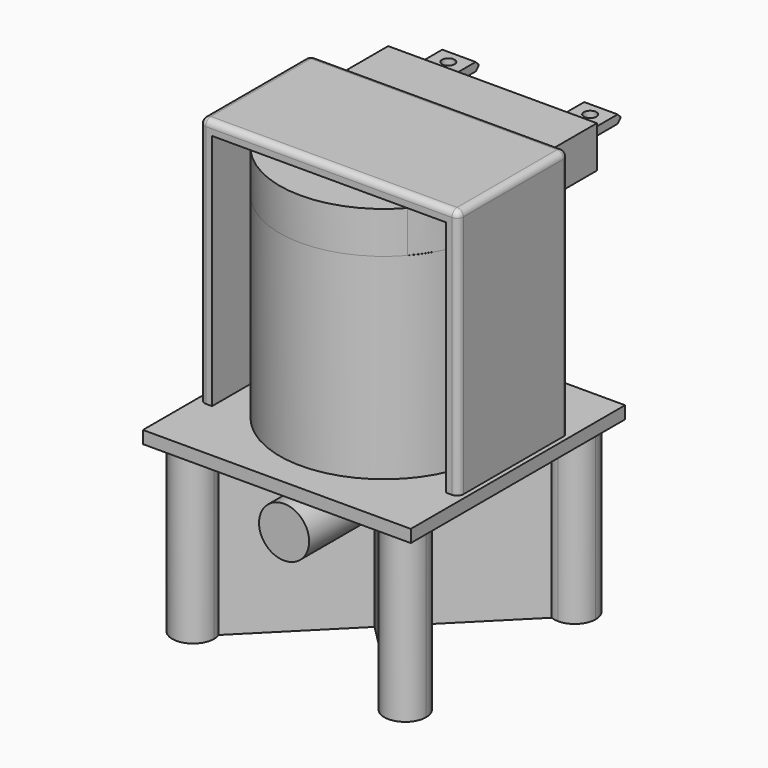
from build123d import *

# Parameters (mm, degrees)
F0_W      = 31
F0_H      = 16.5
F1_DEPTH  = 30
F2_W      = 28
F2_H      = 28.5
F3_DEPTH  = 16.5
F4_R      = 0.762
F5_W      = 28
F5_H      = 24.4999924
F6_DEPTH  = 5
F7_R      = 12.4999974
F8_DEPTH  = 23.5
F10_DEPTH = 5
F11_W     = 2
F11_H     = 0.5
F12_DEPTH = 6
F13_R     = 0.75
F14_DEPTH = 1
F15_SIZE  = 0.4
F16_SIZE  = 0.4
F18_DEPTH = 5
F19_W     = 32.0802
F19_H     = 32.0802
F20_DEPTH = 1.5
F22_DEPTH = 20
F26_DEPTH = 20
F27_R     = 3
F28_DEPTH = 31


# Not quite as in the source:
# - a feature of the source that left no trace in its solid (it failed there, or was rolled back) is left out


with BuildPart() as f1:
    # F0 (on Top) → F1 (new body)
    with BuildSketch(Plane.XY):
        Rectangle(F0_W, F0_H)
    extrude(amount=F1_DEPTH)

    # F2 (on face) → F3 (cut, through all)
    with BuildSketch(Plane.XZ.offset(8.25)):
        with Locations((0, 14.25)):
            Rectangle(F2_W, F2_H)
    extrude(amount=-F3_DEPTH, mode=Mode.SUBTRACT)

    # F4
    f4_edges = [f1.edges().sort_by_distance(p)[0] for p in [
        (15.5, 8.25, 15),
        (0, 8.25, 30),
        (-15.5, 8.25, 15),
        (15.5, 0, 30),
        (15.5, -8.25, 15),
        (0, -8.25, 30),
        (-15.5, 0, 30),
        (-15.5, -8.25, 15),
    ]]
    fillet(f4_edges, radius=F4_R)

    # F5 (on face) → F6 (join)
    with BuildSketch(Plane(origin=(0, 0, 28.5), x_dir=(1, 0, 0), z_dir=(0, 0, -1))):
        with Locations((0, -3.9999962)):
            Rectangle(F5_W, F5_H)
    extrude(amount=F6_DEPTH)

    # F7 (on face) → F8 (join)
    with BuildSketch(Plane(origin=(0, 0, 23.5), x_dir=(1, 0, 0), z_dir=(0, 0, -1))):
        Circle(F7_R)
    extrude(amount=F8_DEPTH)

    # F9 (on face) → F10 (cut)
    with BuildSketch(Plane(origin=(0, 0, 23.5), x_dir=(1, 0, 0), z_dir=(0, 0, -1))):
        with BuildLine():
            add(Edge.make_bspline(
                [(9.3908165247, 8.25), (9.9761542333, 7.5152910471), (11.2114839399, 5.7745359804), (12.1932801678, 3.3671524419), (12.4792695901, 0.7813469518), (12.4999974, 0)],
                knots=[0, 0, 0, 0, 0.3330931337, 0.6537874323, 1, 1, 1, 1], degree=3))
            Line((12.4999974, 0), (12.4999974, -16.2499924))
            Line((12.4999974, -16.2499924), (14, -16.2499924))
            Line((14, -16.2499924), (14, 8.25))
            Line((14, 8.25), (9.3908165247, 8.25))
        make_face()
        with BuildLine():
            add(Edge.make_bspline(
                [(-9.3908165247, 8.25), (-9.8951466827, 7.6039833324), (-10.9690015511, 6.2442324236), (-12.2412171784, 3.3192353758), (-12.4077121811, 1.117573176), (-12.4999974, 0)],
                knots=[0, 0, 0, 0, 0.3063307587, 0.6473537439, 1, 1, 1, 1], degree=3))
            Line((-9.3908165247, 8.25), (-14, 8.25))
            Line((-14, 8.25), (-14, -16.2499924))
            Line((-14, -16.2499924), (-12.4999974, -16.2499924))
            Line((-12.4999974, -16.2499924), (-12.4999974, 0))
        make_face()
    extrude(amount=-F10_DEPTH, mode=Mode.SUBTRACT)

    # F11 (on face) → F12 (join)
    with BuildSketch(Plane(origin=(0, 16.2499924, 0), x_dir=(-1, 0, 0), z_dir=(0, 1, 0))):
        with Locations((-7.4999974, 25.75)):
            Rectangle(F11_W, F11_H)
        with Locations((-7.4999974, 26.25)):
            Rectangle(F11_W, F11_H)
        with Locations((9.4999974, 25.75)):
            Rectangle(F11_W, F11_H)
        with Locations((7.4999974, 25.75)):
            Rectangle(F11_W, F11_H)
        with Locations((9.4999974, 26.25)):
            Rectangle(F11_W, F11_H)
        with Locations((7.4999974, 26.25)):
            Rectangle(F11_W, F11_H)
        with Locations((-9.4999974, 25.75)):
            Rectangle(F11_W, F11_H)
        with Locations((-9.4999974, 26.25)):
            Rectangle(F11_W, F11_H)
    extrude(amount=F12_DEPTH)

    # F13 (on face) → F14 (cut, through all)
    with BuildSketch(Plane.XY.offset(26.5)):
        with Locations((8.4999974, 20.2499924)):
            Circle(F13_R)
        with Locations((-8.4999974, 20.2499924)):
            Circle(F13_R)
    extrude(amount=-F14_DEPTH, mode=Mode.SUBTRACT)

    # F15
    f15_edges = [f1.edges().sort_by_distance(p)[0] for p in [
        (8.499997, 22.249992, 26.5),
        (-8.499997, 22.249992, 26.5),
    ]]
    chamfer(f15_edges, length=F15_SIZE)

    # F16
    f16_edges = [f1.edges().sort_by_distance(p)[0] for p in [
        (8.499997, 22.249992, 25.5),
        (-8.499997, 22.249992, 25.5),
    ]]
    chamfer(f16_edges, length=F16_SIZE)

    # F17 (on face) → F18 (join)
    with BuildSketch(Plane.XY.offset(23.5)):
        with BuildLine():
            Line((9.3908165247, -8.25), (-9.3908165247, -8.25))
            ThreePointArc((-9.3908165247, -8.25), (0, -12.4999974), (9.3908165247, -8.25))
        make_face()
    extrude(amount=F18_DEPTH)

    # F19 (on face) → F20 (join)
    with BuildSketch(Plane(origin=(0, 0, 0), x_dir=(1, 0, 0), z_dir=(0, 0, -1))):
        Rectangle(F19_W, F19_H)
    extrude(amount=F20_DEPTH)

    # F21 (on face) → F22 (join)
    with BuildSketch(Plane(origin=(0, 0, -1.5), x_dir=(1, 0, 0), z_dir=(0, 0, -1))):
        with BuildLine():
            ThreePointArc((-10.2, -12.7), (-10.932233047, -10.932233047), (-12.7, -10.2))
            ThreePointArc((-12.7, -10.2), (-14.467766953, -14.467766953), (-10.2, -12.7))
        make_face()
        with BuildLine():
            ThreePointArc((-12.7, 10.2), (-10.932233047, 10.932233047), (-10.2, 12.7))
            ThreePointArc((-10.2, 12.7), (-14.467766953, 14.467766953), (-12.7, 10.2))
        make_face()
        with BuildLine():
            ThreePointArc((12.7, 10.2), (14.467766953, 10.932233047), (15.2, 12.7))
            ThreePointArc((15.2, 12.7), (12.7, 15.2), (10.2, 12.7))
            ThreePointArc((10.2, 12.7), (10.932233047, 10.932233047), (12.7, 10.2))
        make_face()
        with BuildLine():
            ThreePointArc((15.2, -12.7), (14.467766953, -10.932233047), (12.7, -10.2))
            ThreePointArc((12.7, -10.2), (10.932233047, -10.932233047), (10.2, -12.7))
            ThreePointArc((10.2, -12.7), (12.7, -15.2), (15.2, -12.7))
        make_face()
    extrude(amount=F22_DEPTH)


with BuildPart() as f26:
    # F25 (on face) → F26 (new body)
    with BuildSketch(Plane(origin=(0, 0, -21.5), x_dir=(1, 0, 0), z_dir=(0, 0, -1))):
        with BuildLine():
            ThreePointArc((-11.7690392124, -10.379803454), (-10.9186518108, -10.945919435), (-10.3657199255, -11.8049376927))
            Line((-10.3657199255, -11.8049376927), (-3.5923e-06, -1.4158147652))
            Line((-3.5923e-06, -1.4158147652), (1.4126173591, -4.0058e-06))
            Line((1.4126173591, -4.0058e-06), (11.7690392124, 10.379803454))
            ThreePointArc((11.7690392124, 10.379803454), (10.9186518108, 10.945919435), (10.3657199255, 11.8049376927))
            Line((10.3657199255, 11.8049376927), (0, 1.4158111649))
            Line((0, 1.4158111649), (-1.4126177626, 3.6014e-06))
            Line((-1.4126177626, 3.6014e-06), (-11.7690392124, -10.379803454))
        make_face()
        with BuildLine():
            Line((1.4126173591, -4.0058e-06), (-3.5923e-06, -1.4158147652))
            Line((-3.5923e-06, -1.4158147652), (10.3664711716, -11.8029809328))
            ThreePointArc((10.3664711716, -11.8029809328), (10.9201168847, -10.9444328279), (11.7709684555, -10.3790302912))
            Line((11.7709684555, -10.3790302912), (1.4126173591, -4.0058e-06))
        make_face()
        with BuildLine():
            Line((-11.7709690322, 10.3790300603), (-1.4126177626, 3.6014e-06))
            Line((-1.4126177626, 3.6014e-06), (0, 1.4158111649))
            Line((0, 1.4158111649), (-10.3664731696, 11.8029757351))
            ThreePointArc((-10.3664731696, 11.8029757351), (-10.920119058, 10.9444306245), (-11.7709690322, 10.3790300603))
        make_face()
    extrude(amount=-F26_DEPTH)


with BuildPart() as f28:
    # F27 (on face) → F28 (new body)
    with BuildSketch(Plane(origin=(0, 16.0401, 0), x_dir=(-1, 0, 0), z_dir=(0, 1, 0))):
        with Locations((0, -6)):
            Circle(F27_R)
    extrude(amount=-F28_DEPTH)


solid = Compound([f1.part, f26.part, f28.part])
